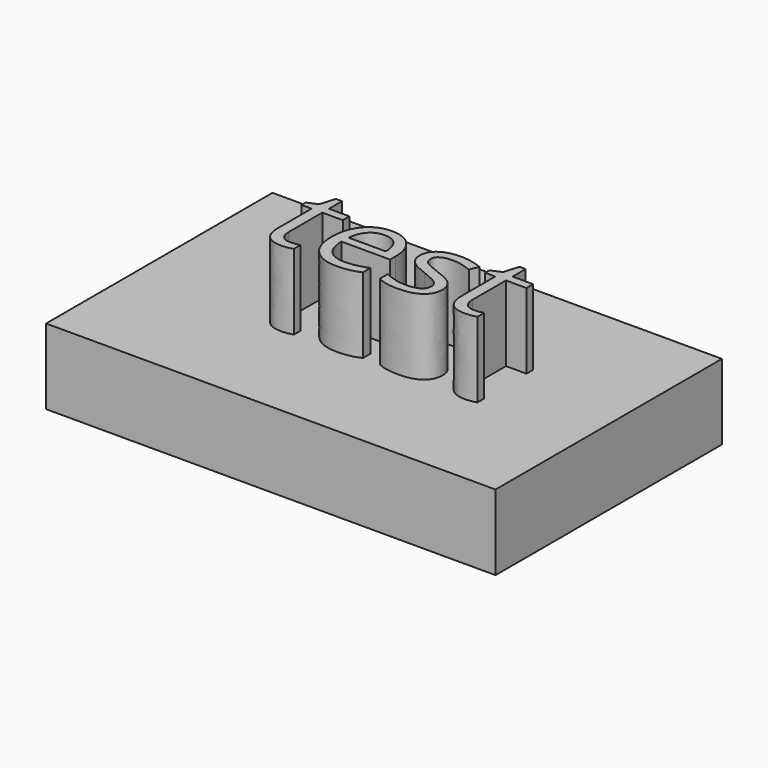
from build123d import *

# Parameters (mm, degrees)
F0_W         = 148.969758302
F0_H         = 93.8017144799
F1_DEPTH     = 25
F2_TEXT_SIZE = 43.7621001361
F3_DEPTH     = 25


# Not quite as in the source:
# - a feature names something its author has since deleted; it is built from what else it names
# - Text() gives the source's letters only with a copy of the font that has no kerning and outlines rounded to 1/6400 em; it was checked with that copy


with BuildPart() as f1:
    # F0 (on Top) → F1 (new body)
    with BuildSketch(Plane.XY):
        with Locations((12.6391928643, -9.8100416362)):
            Rectangle(F0_W, F0_H)
    extrude(amount=F1_DEPTH)

    # F2 (on face) → F3 (join)
    with BuildSketch(Plane.XY.offset(25)):
        with Locations((-22.4142484367, -21.6820742935)):
            Text('test', F2_TEXT_SIZE, font='Open Sans', text_align=(TextAlign.LEFT, TextAlign.BOTTOM))
    extrude(amount=F3_DEPTH)


solid = f1.part
